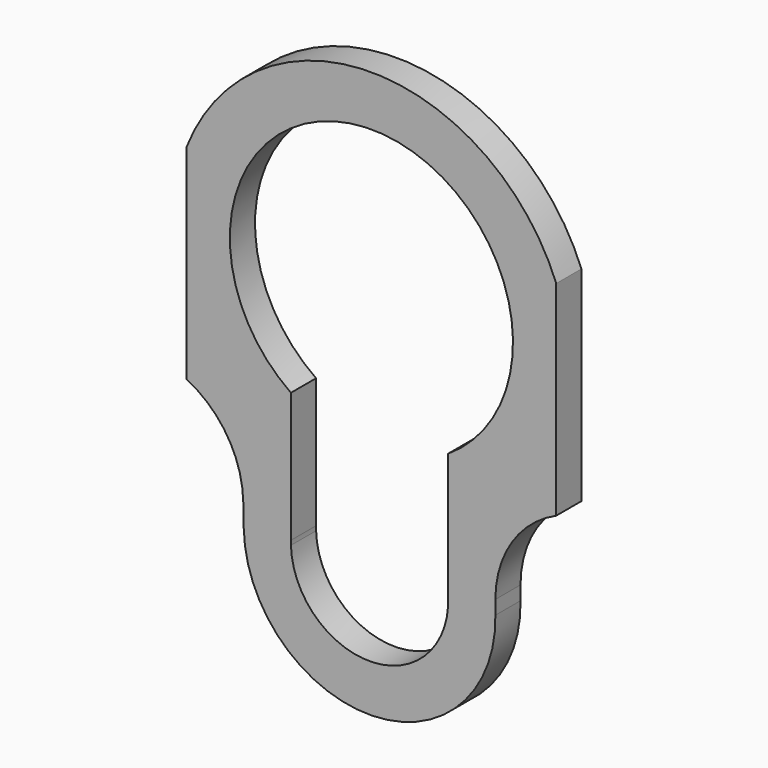
from build123d import *

# Parameters (mm, degrees)
F1_DEPTH    = 2
F2_T1_DEPTH = 2


# Not quite as in the source:
# - a fillet or chamfer that OpenCascade refuses, or shapes differently, is made with other operations: its cross-section is extruded or revolved along the edge and cut away or added


with BuildPart() as f1:
    # F0 (on Front) → F1 (new body)
    with BuildSketch(Plane.XZ):
        with BuildLine():
            Line((-11.6313876303, 13), (-11.6313876303, 0))
            Line((-11.6313876303, 0), (-8.150026169, 0))
            Line((-8.150026169, 0), (-7.9982068951, -7.1693707857))
            ThreePointArc((-7.9982068951, -7.1693707857), (0.1698610087, -14.9981964991), (7.998186073, -6.829648769))
            Line((7.998186073, -6.829648769), (7.998186073, 0))
            Line((7.998186073, 0), (11.8686123697, 0))
            Line((11.8686123697, 0), (11.8686123697, 13))
            ThreePointArc((11.8686123697, 13), (0.1186123697, 21), (-11.6313876303, 13))
        make_face()
        with BuildLine():
            ThreePointArc((-4.9980202119, -7.1406910146), (-5, -7), (-4.9980202119, -6.8593089854))
            Line((-4.9980202119, -6.8593089854), (-4.9980202119, 1.395497035))
            ThreePointArc((-4.9980202119, 1.395497035), (0.2650718597, 17.7983630087), (4.9915903324, 1.2329118096))
            Line((4.9915903324, 1.2329118096), (4.9915903324, -6.7101276944))
            ThreePointArc((4.9915903324, -6.7101276944), (0.2153056642, -11.9953621962), (-4.9980202119, -7.1406910146))
        make_face(mode=Mode.SUBTRACT)
    extrude(amount=F1_DEPTH)

    # F2: fillet of radius 6.5 on 2 edges, made by hand

    # F2_s2 → F2_t1 (join)
    with BuildSketch(Plane.XZ):
        with BuildLine():
            ThreePointArc((-11.6313876303, 0), (-9.0385133393, -2.3384510594), (-8.029721431, -5.6811579463))
            Line((-8.029721431, -5.6811579463), (-8.150026169, 0))
            Line((-8.150026169, 0), (-11.6313876303, 0))
        make_face()
        with BuildLine():
            ThreePointArc((7.998186073, -5.9443538033), (9.0510662344, -2.3976813538), (11.8686123697, 0))
            Line((11.8686123697, 0), (7.998186073, 0))
            Line((7.998186073, 0), (7.998186073, -5.9443538033))
        make_face()
    extrude(amount=F2_T1_DEPTH)


solid = f1.part
